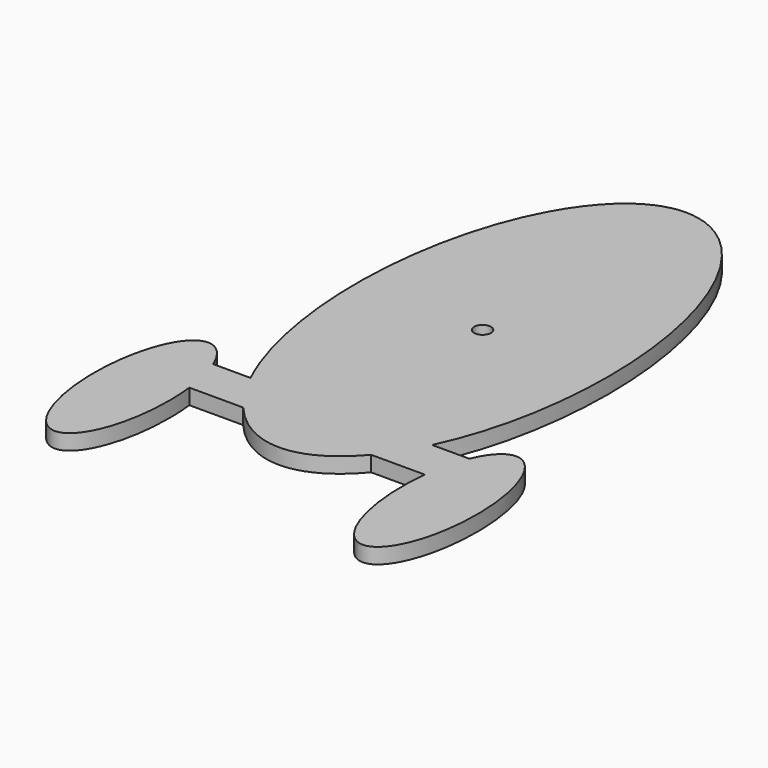
from build123d import *

# Parameters (mm, degrees)
F1_DEPTH = 7


with BuildPart() as f1:
    # F0 (on Top) → F1 (new body)
    with BuildSketch(Plane.XY):
        with BuildLine():
            add(Edge.make_bspline(
                [(41.0325361716, -79.8311173649), (92.2831646624, 27.3740003908), (27.9046112087, 100.2799772001), (-36.473942245, 173.1859540094), (-55.1512876885, 29.0929770047), (-73.8286331319, -115), (0, -115)],
                knots=[0.8035112137, 0.8035112137, 0.8035112137, 2.6300692449, 2.6300692449, 4.456627276, 4.456627276, 6.2831853072, 6.2831853072, 6.2831853072], degree=2, weights=[1, 0.6111536596, 1, 0.6111536596, 1, 0.6111536596, 1]))
            add(Edge.make_bspline(
                [(0, -115), (15.5169707114, -115), (28.8931550214, -99.1341173649)],
                knots=[0, 0, 0, 0.5315236702, 0.5315236702, 0.5315236702], degree=2, weights=[1, 0.9648926892, 1]))
            Line((28.8931550214, -99.1341173649), (14.8503418565, -99.1341173649))
            Line((14.8503418565, -99.1341173649), (14.8503418565, -79.8311173649))
            Line((14.8503418565, -79.8311173649), (41.0325361716, -79.8311173649))
        make_face()
        with BuildLine():
            ThreePointArc((3.8, 0), (2.6870057685, -2.6870057685), (0, -3.8))
            ThreePointArc((0, -3.8), (-2.6870057685, 2.6870057685), (3.8, 0))
        make_face(mode=Mode.SUBTRACT)
        with BuildLine():
            Line((14.8503418565, -99.1341173649), (28.8931550214, -99.1341173649))
            add(Edge.make_bspline(
                [(28.8931550214, -99.1341173649), (35.6175159706, -91.1581565719), (41.0325361716, -79.8311173649)],
                knots=[0.5315236702, 0.5315236702, 0.5315236702, 0.8035112137, 0.8035112137, 0.8035112137], degree=2, weights=[1, 0.9907670899, 1]))
            Line((41.0325361716, -79.8311173649), (14.8503418565, -79.8311173649))
            Line((14.8503418565, -79.8311173649), (14.8503418565, -99.1341173649))
        make_face()
        with BuildLine():
            add(Edge.make_bspline(
                [(28.8931550214, -99.1341173649), (35.6175159706, -91.1581565719), (41.0325361716, -79.8311173649)],
                knots=[0.5315236702, 0.5315236702, 0.5315236702, 0.8035112137, 0.8035112137, 0.8035112137], degree=2, weights=[1, 0.9907670899, 1]))
            Line((28.8931550214, -99.1341173649), (53.2561757529, -99.1341173649))
            add(Edge.make_bspline(
                [(57.9107478758, -79.8311173649), (54.5561014443, -87.8810002796), (53.2561757529, -99.1341173649)],
                knots=[3.8980546745, 3.8980546745, 3.8980546745, 4.4267019246, 4.4267019246, 4.4267019246], degree=2, weights=[1, 0.965269429, 1]))
            Line((57.9107478758, -79.8311173649), (41.0325361716, -79.8311173649))
        make_face()
        with BuildLine():
            Line((66.8503418565, -99.1341173649), (53.2561757529, -99.1341173649))
            add(Edge.make_bspline(
                [(53.2561757529, -99.1341173649), (46.8397172233, -154.6797224603), (69.6079134941, -154.6797224603)],
                knots=[4.4267019246, 4.4267019246, 4.4267019246, 6.2831853072, 6.2831853072, 6.2831853072], degree=2, weights=[1, 0.5992425527, 1]))
            add(Edge.make_bspline(
                [(69.6079134941, -154.6797224603), (94.7186627471, -154.6797224603), (85.4458382886, -95.3441536003), (76.1730138301, -36.0085847403), (57.9107478758, -79.8311173649)],
                knots=[0, 0, 0, 1.9490273372, 1.9490273372, 3.8980546745, 3.8980546745, 3.8980546745], degree=2, weights=[1, 0.5615705246, 1, 0.5615705246, 1]))
            Line((57.9107478758, -79.8311173649), (66.8503418565, -79.8311173649))
            Line((66.8503418565, -79.8311173649), (66.8503418565, -99.1341173649))
        make_face()
        with BuildLine():
            add(Edge.make_bspline(
                [(57.9107478758, -79.8311173649), (54.5561014443, -87.8810002796), (53.2561757529, -99.1341173649)],
                knots=[3.8980546745, 3.8980546745, 3.8980546745, 4.4267019246, 4.4267019246, 4.4267019246], degree=2, weights=[1, 0.965269429, 1]))
            Line((53.2561757529, -99.1341173649), (66.8503418565, -99.1341173649))
            Line((66.8503418565, -99.1341173649), (66.8503418565, -79.8311173649))
            Line((66.8503418565, -79.8311173649), (57.9107478758, -79.8311173649))
        make_face()
        with BuildLine():
            add(Edge.make_bspline(
                [(-57.9107478758, -79.8311173649), (-76.1730138301, -36.0085847403), (-85.4458382886, -95.3441536003), (-94.7186627471, -154.6797224603), (-69.6079134941, -154.6797224603)],
                knots=[2.3851306327, 2.3851306327, 2.3851306327, 4.3341579699, 4.3341579699, 6.2831853072, 6.2831853072, 6.2831853072], degree=2, weights=[1, 0.5615705246, 1, 0.5615705246, 1]))
            add(Edge.make_bspline(
                [(-69.6079134941, -154.6797224603), (-46.8397172233, -154.6797224603), (-53.2561757529, -99.1341173649)],
                knots=[0, 0, 0, 1.8564833826, 1.8564833826, 1.8564833826], degree=2, weights=[1, 0.5992425527, 1]))
            Line((-53.2561757529, -99.1341173649), (-66.8503418565, -99.1341173649))
            Line((-66.8503418565, -99.1341173649), (-66.8503418565, -79.8311173649))
            Line((-66.8503418565, -79.8311173649), (-57.9107478758, -79.8311173649))
        make_face()
        with BuildLine():
            Line((-66.8503418565, -99.1341173649), (-53.2561757529, -99.1341173649))
            add(Edge.make_bspline(
                [(-53.2561757529, -99.1341173649), (-54.5561014443, -87.8810002796), (-57.9107478758, -79.8311173649)],
                knots=[1.8564833826, 1.8564833826, 1.8564833826, 2.3851306327, 2.3851306327, 2.3851306327], degree=2, weights=[1, 0.965269429, 1]))
            Line((-57.9107478758, -79.8311173649), (-66.8503418565, -79.8311173649))
            Line((-66.8503418565, -79.8311173649), (-66.8503418565, -99.1341173649))
        make_face()
        with BuildLine():
            add(Edge.make_bspline(
                [(-53.2561757529, -99.1341173649), (-54.5561014443, -87.8810002796), (-57.9107478758, -79.8311173649)],
                knots=[1.8564833826, 1.8564833826, 1.8564833826, 2.3851306327, 2.3851306327, 2.3851306327], degree=2, weights=[1, 0.965269429, 1]))
            Line((-53.2561757529, -99.1341173649), (-14.8503418565, -99.1341173649))
            Line((-14.8503418565, -99.1341173649), (-14.8503418565, -79.8311173649))
            Line((-14.8503418565, -79.8311173649), (-57.9107478758, -79.8311173649))
        make_face()
    extrude(amount=F1_DEPTH)


solid = f1.part
